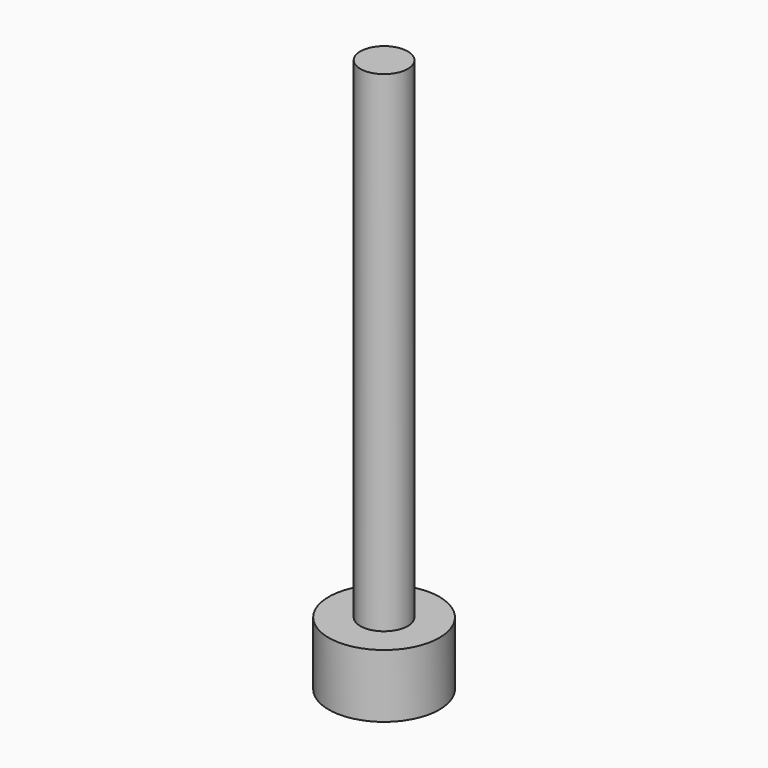
from build123d import *

# Parameters (mm, degrees)
F0_R     = 1.5
F1_DEPTH = 35
F0_R_2   = 3.5
F2_DEPTH = 4


# Not quite as in the source:
# - a feature names something its author has since deleted; it is built from what else it names


with BuildPart() as f1:
    # F0 (on Top) → F1 (new body)
    with BuildSketch(Plane.XY):
        Circle(F0_R)
    extrude(amount=F1_DEPTH)

    # F0 (on Top) → F2 (join)
    with BuildSketch(Plane.XY):
        Circle(F0_R_2)
        Circle(F0_R, mode=Mode.SUBTRACT)
    extrude(amount=F2_DEPTH)


solid = f1.part
